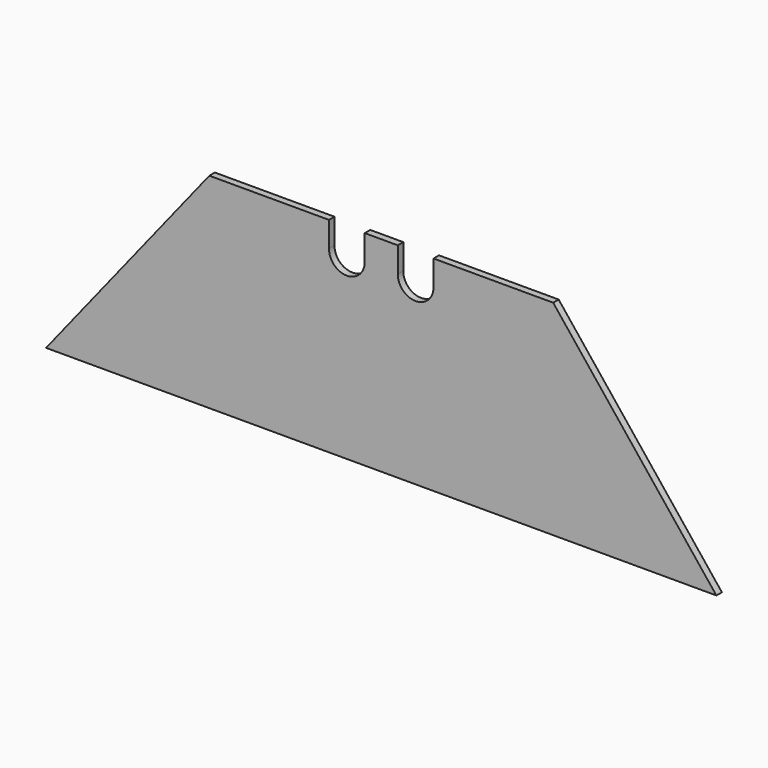
from build123d import *

# Parameters (mm, degrees)
F1_DEPTH      = 0.3175
F3_DEPTH      = 0.3185
F3_DEPTH_BACK = 0.3185


with BuildPart() as f1:
    # F0 (on Front) → F1 (new body, symmetric)
    with BuildSketch(Plane.XZ):
        Polygon((15.875, 0), (-15.875, 0), (-30.95, -18.9), (30.95, -18.9), align=None)
    extrude(amount=F1_DEPTH, both=True)

    # F2 (on Front) → F3 (cut, two sides)
    with BuildSketch(Plane.XZ) as f3_sk:
        with BuildLine():
            Line((-1.525, 0), (-4.825, 0))
            Line((-4.825, 0), (-4.825, -2.35))
            ThreePointArc((-4.825, -2.35), (-3.175, -4), (-1.525, -2.35))
            Line((-1.525, -2.35), (-1.525, 0))
        make_face()
        with BuildLine():
            Line((4.825, -2.35), (4.825, 0))
            Line((4.825, 0), (1.525, 0))
            Line((1.525, 0), (1.525, -2.35))
            ThreePointArc((1.525, -2.35), (3.175, -4), (4.825, -2.35))
        make_face()
    extrude(amount=-F3_DEPTH, mode=Mode.SUBTRACT)
    extrude(f3_sk.sketch, amount=F3_DEPTH_BACK, mode=Mode.SUBTRACT)


solid = f1.part
